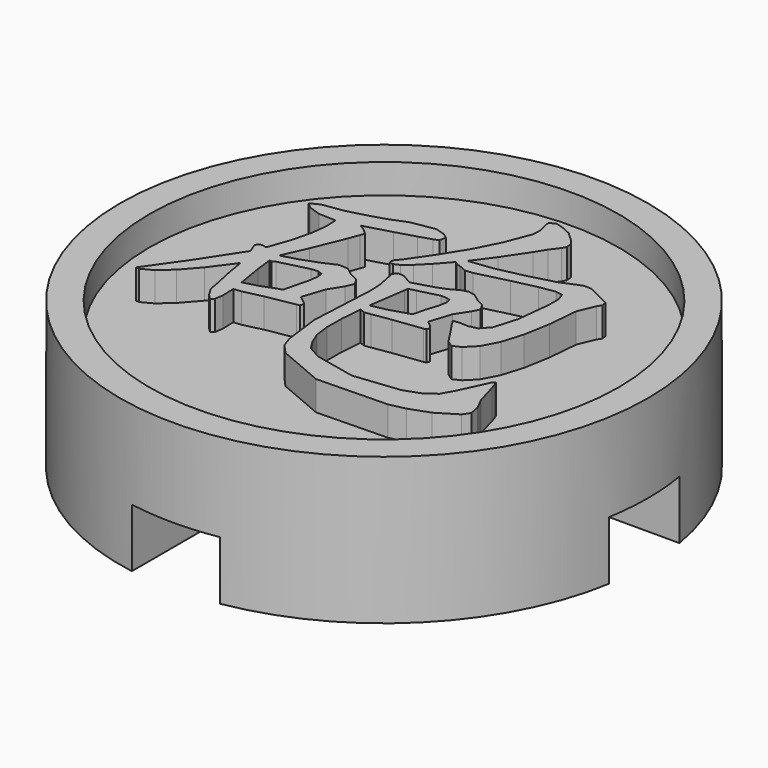
from build123d import *

# Parameters (mm, degrees)
F0_R     = 9
F1_DEPTH = 4
F3_W     = 3
F3_H     = 3
F4_DEPTH = 2
F2_R     = 9
F2_R_2   = 8
F5_DEPTH = 1
F7_DEPTH = 1


# Not quite as in the source:
# - a feature names something its author has since deleted; it is built from what else it names


with BuildPart() as f1:
    # F0 (on Top) → F1 (new body)
    with BuildSketch(Plane.XY):
        with Locations((-31.3306450844, 19.7580661625)):
            Circle(F0_R)
    extrude(amount=F1_DEPTH)

    # F3 (on face) → F4 (cut)
    with BuildSketch(Plane(origin=(0, 0, 0), x_dir=(1, 0, 0), z_dir=(0, 0, -1))):
        with BuildLine():
            ThreePointArc((-32.8306450844, -28.6321858371), (-32.0832814269, -28.7265408676), (-31.3306450844, -28.7580661625))
            ThreePointArc((-31.3306450844, -28.7580661625), (-30.5780087419, -28.7265408676), (-29.8306450844, -28.6321858371))
            Line((-29.8306450844, -28.6321858371), (-29.8306450844, -21.2580661625))
            Line((-29.8306450844, -21.2580661625), (-32.8306450844, -21.2580661625))
            Line((-32.8306450844, -21.2580661625), (-32.8306450844, -28.6321858371))
        make_face()
        with BuildLine():
            ThreePointArc((-40.204764759, -18.2580661625), (-40.2991197895, -19.0054298199), (-40.3306450844, -19.7580661625))
            ThreePointArc((-40.3306450844, -19.7580661625), (-40.2991197895, -20.510702505), (-40.204764759, -21.2580661625))
            Line((-40.204764759, -21.2580661625), (-32.8306450844, -21.2580661625))
            Line((-32.8306450844, -21.2580661625), (-32.8306450844, -18.2580661625))
            Line((-32.8306450844, -18.2580661625), (-40.204764759, -18.2580661625))
        make_face()
        with Locations((-31.3306450844, -19.7580661625)):
            Rectangle(F3_W, F3_H)
        with BuildLine():
            Line((-29.8306450844, -18.2580661625), (-29.8306450844, -21.2580661625))
            Line((-29.8306450844, -21.2580661625), (-22.4565254097, -21.2580661625))
            ThreePointArc((-22.4565254097, -21.2580661625), (-22.3621703793, -20.510702505), (-22.3306450844, -19.7580661625))
            ThreePointArc((-22.3306450844, -19.7580661625), (-22.3621703793, -19.0054298199), (-22.4565254097, -18.2580661625))
            Line((-22.4565254097, -18.2580661625), (-29.8306450844, -18.2580661625))
        make_face()
        with BuildLine():
            Line((-32.8306450844, -10.8839464878), (-32.8306450844, -18.2580661625))
            Line((-32.8306450844, -18.2580661625), (-29.8306450844, -18.2580661625))
            Line((-29.8306450844, -18.2580661625), (-29.8306450844, -10.8839464878))
            ThreePointArc((-29.8306450844, -10.8839464878), (-30.5780087419, -10.7895914574), (-31.3306450844, -10.7580661625))
            ThreePointArc((-31.3306450844, -10.7580661625), (-32.0832814269, -10.7895914574), (-32.8306450844, -10.8839464878))
        make_face()
    extrude(amount=-F4_DEPTH, mode=Mode.SUBTRACT)

    # F2 (on face) → F5 (join)
    with BuildSketch(Plane.XY.offset(4)):
        with Locations((-31.3306450844, 19.7580661625)):
            Circle(F2_R)
        with Locations((-31.3306450844, 19.7580661625)):
            Circle(F2_R_2, mode=Mode.SUBTRACT)
    extrude(amount=F5_DEPTH)

    # F6 (on face) → F7 (join)
    with BuildSketch(Plane.XY.offset(4)):
        Polygon((-34.8750185671, 17.3237123537), (-34.8894101453, 17.7809921533), (-34.6251999422, 17.808091581), (-33.9867103865, 17.957974153), (-33.012882311, 18.1332601341), (-32.915508721, 18.1535939224), (-32.8672520756, 18.2789149495), (-32.9722393144, 18.3762946845), (-33.1958065208, 18.5431067176), (-32.9451398866, 19.300151661), (-32.657234583, 19.7625072264), (-32.5454571248, 20.030945186), (-32.6707842969, 20.2468864537), (-32.9510820968, 20.3857571947), (-33.2364495175, 20.6025341817), (-33.5506123845, 20.6279437358), (-34.0087340484, 20.4196345518), (-34.563393583, 20.2180971523), (-35.1400583445, 20.05043711), (-34.7683168747, 20.8853698645), (-34.3237449247, 21.9675649259), (-34.196727879, 22.3130979922), (-34.1408452949, 22.4654938671), (-34.3279911163, 22.6331907794), (-34.5202127034, 22.7534483307), (-33.6090328516, 23.01000187), (-32.9417601394, 23.207317658), (-32.5234334629, 23.3402338989), (-32.3557734205, 23.407152894), (-32.3151304239, 23.6307078104), (-32.498871918, 23.760244304), (-32.8164391123, 23.8542627269), (-33.615816926, 23.7222067853), (-34.1654068397, 23.5019701661), (-34.7200417944, 23.3292343579), (-35.3957945995, 23.1513982039), (-36.1088106541, 23.0447210915), (-36.4068859244, 22.8922637667), (-36.2273598968, 22.7297286501), (-35.8115833932, 22.5899914649), (-35.2315143044, 22.5705118309), (-35.2154328526, 22.1632215653), (-35.2764096376, 21.6381931963), (-35.4322098396, 20.9895275289), (-35.7023438179, 20.2096170593), (-35.7658523407, 20.2104650686), (-35.7937997778, 20.2333367398), (-35.9292846265, 20.2333367398), (-35.9800914448, 20.2096170593), (-36.0292083895, 20.1046298205), (-35.9665478759, 19.9454252912), (-35.8987993066, 19.7760569402), (-36.7896392251, 18.4144059432), (-37.6330557597, 17.2153207877), (-37.6889444888, 17.1365849674), (-37.5788605911, 17.1238832628), (-37.2003387339, 17.324560363), (-36.7625397974, 17.7098638367), (-36.2671610291, 18.2738207487), (-35.7158935317, 19.013936231), (-35.7252031991, 19.0257960712), (-35.6752443901, 19.0782989081), (-35.5736307535, 18.4736744196), (-35.4279882281, 17.7809921533), (-35.3593977944, 17.4041626277), (-35.1773215939, 17.1103335489), (-35.0189589289, 16.9502810103), (-34.9165095731, 17.0324211579), align=None)
        Polygon((-33.8876407778, 18.5490489277), (-33.9172780885, 18.5532766842), (-34.4863292013, 18.3424111823), (-34.9537728225, 18.2145522723), (-35.0985611936, 19.1045503266), (-35.16377188, 19.6710697014), (-35.085859489, 19.6651274913), (-34.9808722502, 19.7218580847), (-33.9850205129, 19.9725247189), (-33.7504660554, 19.991992063), (-33.6022733571, 19.9318755773), (-33.5726360464, 19.7641971), (-33.615816926, 19.4339527811), (-33.7250565013, 19.0012345264), (-33.8258159836, 18.580376112), align=None, mode=Mode.SUBTRACT)
        Polygon((-31.6520793233, 22.2258390639), (-31.2278165816, 22.7026292224), (-31.1439988505, 22.6204706399), (-31.0042616652, 22.5840922697), (-30.7409486314, 22.4663541664), (-30.4792332963, 22.4925932948), (-29.4122778223, 22.7584872265), (-28.6061159342, 22.943082875), (-28.077707818, 23.0269620561), (-27.8440136599, 22.990522236), (-27.7550955829, 22.7322480981), (-27.752514685, 22.3232372339), (-27.8787328814, 21.1614644878), (-28.108186993, 20.3789915552), (-28.3758015233, 20.078378402), (-28.6705154813, 20.0131738606), (-28.9719274838, 20.0233376822), (-29.1811031121, 20.0030038939), (-29.0634264587, 19.8133201897), (-28.7577129597, 19.358596708), (-28.5281973982, 19.0003865171), (-28.3046424817, 18.8471241979), (-28.0404691486, 18.9732932344), (-27.7008967274, 19.3137013749), (-27.4206235075, 19.8505834391), (-27.2013086376, 20.5695232688), (-27.0446112662, 21.4561169958), (-26.9540340406, 22.4782140067), (-26.716038386, 23.0447210915), (-26.6254611604, 23.1886983233), (-26.6483205416, 23.3428147968), (-26.9193148191, 23.4867305786), (-27.4375222436, 23.7492447631), (-27.7118962684, 23.7552054082), (-27.9354511848, 23.671387677), (-28.3885216628, 23.4791722348), (-29.1819634114, 23.2648962608), (-30.1667603028, 23.0455813908), (-31.0313610929, 22.9397031278), (-30.5342924511, 23.6112281764), (-29.9847455523, 24.4301102041), (-29.7586097379, 24.7934023058), (-29.5376357194, 25.0871945146), (-29.4639572299, 25.2235519526), (-29.4834368639, 25.4157673948), (-29.6349724394, 25.6028824912), (-29.9305466968, 25.8764576665), (-30.2793980603, 26.0339538872), (-30.5436328434, 26.100012583), (-30.7172289509, 25.9814141804), (-30.675688785, 25.7714397028), (-30.6113506878, 25.488585585), (-30.6249311266, 25.2328923449), (-30.9602635013, 24.363191209), (-31.3700732148, 23.5527892744), (-31.8832540335, 22.7246283043), (-32.4472355254, 21.9032268287), (-32.5742464262, 21.7711708872), (-32.6064216197, 21.6661529234), (-32.5894860137, 21.5696150527), (-32.4607852393, 21.5611349596), (-32.2829613753, 21.6415729436), (-32.0077331963, 21.867647308), align=None)
        Polygon((-30.7400883321, 21.2190430905), (-31.4649519369, 21.0090071629), (-31.8036517689, 21.2054626516), (-31.976406012, 21.2283220329), (-32.0678681169, 21.1919436627), (-32.134768677, 21.0716861115), (-32.0949675447, 20.917563493), (-31.9967213653, 20.4196345518), (-31.976406012, 19.9725247189), (-32.0907152082, 17.7352733908), (-31.9357630154, 16.4938492201), (-31.8061896518, 16.1093999007), (-31.5021906064, 15.7723715075), (-29.9203460051, 15.100012583), (-27.5154407797, 15.1559006976), (-26.9768934218, 15.2744542418), (-26.2986088787, 15.518331271), (-25.6253632315, 15.9281839995), (-25.4721070573, 16.1559728175), (-25.5339257066, 16.4938492201), (-25.7422410356, 16.9113278873), (-25.9539361117, 17.6488870518), (-26.0064143687, 17.8089334453), (-26.0589540755, 17.9368169353), (-26.1410512081, 17.8893837193), (-26.2045904559, 17.7403430117), (-26.5712623049, 16.9485849917), (-26.8210563498, 16.4938492201), (-27.1928285446, 16.2245693962), (-27.752514685, 16.0230258517), (-29.3064610092, 15.8536697907), (-30.6892692238, 16.151745061), (-31.1397588039, 16.4023932602), (-31.3463535343, 16.7309599954), (-31.5005314577, 17.1094855396), (-31.5665901535, 17.6150219846), (-31.5614898077, 18.2391138171), (-31.5021906064, 18.9732932344), (-31.323555603, 18.905544665), (-31.109279629, 18.93602384), (-30.4800935956, 19.0359598929), (-29.5105362916, 19.1595910464), (-29.4207579153, 19.1824442826), (-29.3784189001, 19.2882979657), (-29.4732361722, 19.3966895317), (-29.656172672, 19.5525081688), (-29.4173781681, 20.2892193239), (-29.1311443031, 20.7346454282), (-29.0083673039, 20.9700478949), (-29.1311443031, 21.1919436627), (-29.3733185543, 21.3172401099), (-29.6696916609, 21.5340355319), (-29.8992072225, 21.5755142478), (-30.1032825049, 21.520455093), (-30.4140348998, 21.3477192848), align=None)
        Polygon((-31.4649519369, 19.3018476796), (-31.2786356899, 20.5754408989), (-31.2650552511, 20.6939962866), (-31.020361552, 20.7558210808), (-30.3335969158, 20.9310886269), (-30.1286613341, 20.9260190061), (-29.9982645412, 20.8904640653), (-29.9661262175, 20.7219375786), (-30.0219842217, 20.4331842657), (-30.1498615667, 20.0351729425), (-30.2455391381, 19.6304205598), (-30.3107375346, 19.6033211321), (-30.3234576742, 19.6033211321), (-30.9450239138, 19.4119291192), align=None, mode=Mode.SUBTRACT)
    extrude(amount=F7_DEPTH)


solid = f1.part
